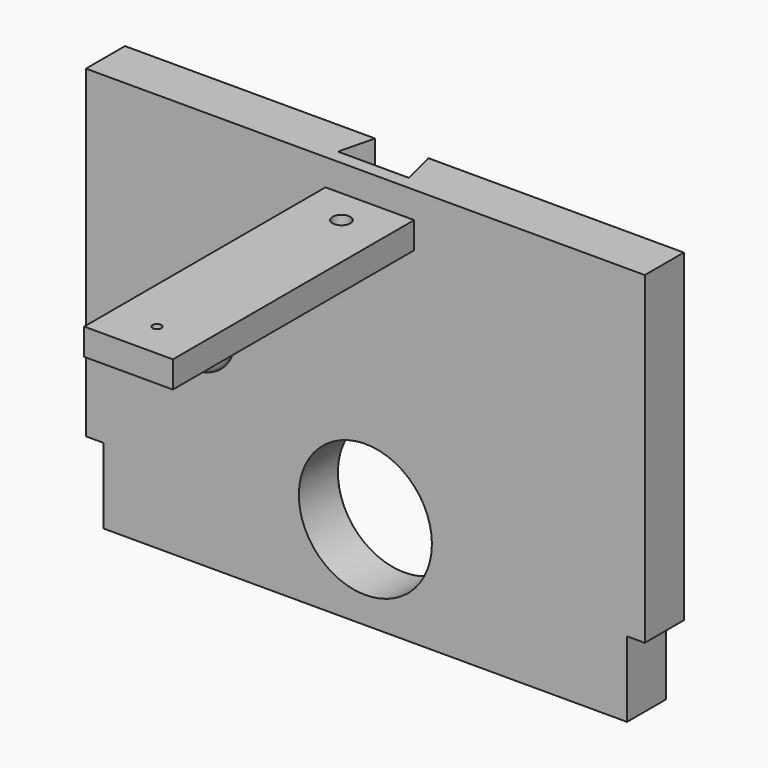
from build123d import *

# Parameters (mm, degrees)
F0_R      = 7.5
F1_DEPTH  = 5.5
F3_DEPTH  = 25
F4_W      = 10
F4_H      = 3
F5_DEPTH  = 34
F6_R      = 0.5
F7_DEPTH  = 6
F6_R_2    = 1
F8_DEPTH  = 25
F9_R      = 0.75
F10_ANGLE = 180


# Not quite as in the source:
# - a feature names something its author has since deleted; it is built from what else it names


with BuildPart() as f1:
    # F0 (on Front) → F1 (new body)
    with BuildSketch(Plane.XZ):
        Polygon((0, 8.5), (0, 0), (59, 0), (59, 8.5), (61, 8.5), (61, 45), (-2, 45), (-2, 8.5), align=None)
        with Locations((29.5, 10.5)):
            Circle(F0_R, mode=Mode.SUBTRACT)
    extrude(amount=F1_DEPTH)

    # F2 (on face) → F3 (cut)
    with BuildSketch(Plane.XY.offset(45)):
        Polygon((26.2, 0), (25.2, -4), (33.2, -4), (32.2, 0), align=None)
    extrude(amount=-F3_DEPTH, mode=Mode.SUBTRACT)

    # F4 (on face) → F5 (join)
    with BuildSketch(Plane.XZ.offset(5.5)):
        with Locations((30, 40.5)):
            Rectangle(F4_W, F4_H)
    extrude(amount=F5_DEPTH)

    # F6 (on face) → F7 (cut)
    with BuildSketch(Plane.XY.offset(42)):
        with Locations((30, -35.5)):
            Circle(F6_R)
    extrude(amount=-F7_DEPTH, mode=Mode.SUBTRACT)

    # F6 (on face) → F8 (cut)
    with BuildSketch(Plane.XY.offset(42)):
        with Locations((30, -9.5)):
            Circle(F6_R_2)
    extrude(amount=-F8_DEPTH, mode=Mode.SUBTRACT)

    # F9 (on face) → F10 (revolve)
    with BuildSketch(Plane(origin=(0, 0, 39), x_dir=(1, 0, 0), z_dir=(0, 0, -1))):
        with Locations((33, 29.5)):
            Circle(F9_R)
    revolve(axis=Axis((30, -12.9445128906, 39), (0, 1, 0)), revolution_arc=F10_ANGLE)


solid = f1.part
